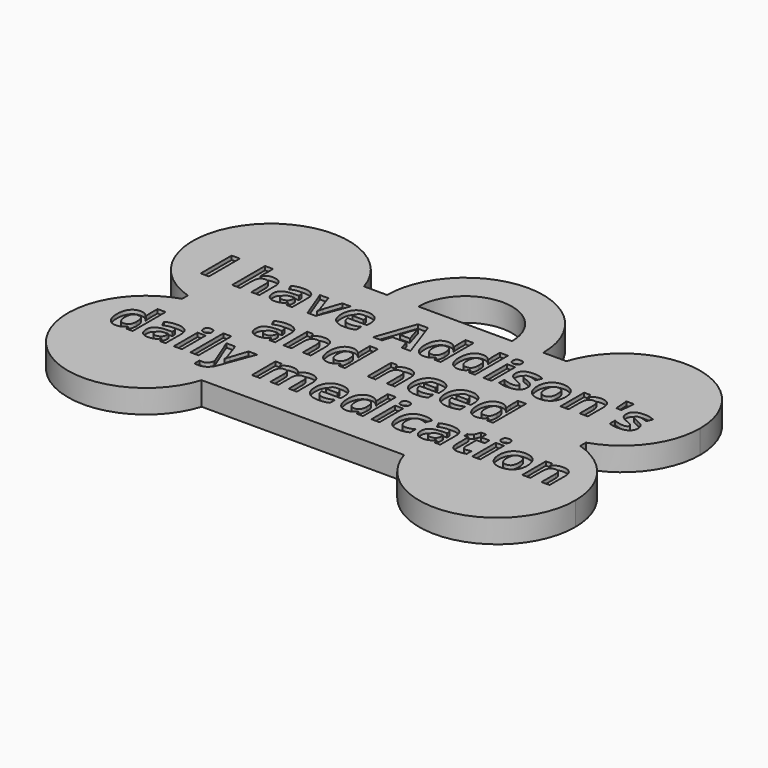
from build123d import *

# Parameters (mm, degrees)
F0_W          = 45
F0_H          = 20
F1_DEPTH      = 3
F3_DEPTH      = 3
F4_W          = 51
F4_H          = 26
F5_DEPTH      = 3
F6_R          = 10
F6_R_2        = 6
F7_DEPTH      = 3
F8_TEXT_SIZE  = 6.9444444444
F9_DEPTH      = 0.5
F10_TEXT_SIZE = 6.9444444444
F11_DEPTH     = 0.5


# Not quite as in the source:
# - Text() gives the source's letters only with a copy of the font that has no kerning and outlines rounded to 1/6400 em; it was checked with that copy


with BuildPart() as f1:
    # F0 (on Top) → F1 (new body)
    with BuildSketch(Plane.XY):
        with Locations((6.4884250968, 4.8540276475)):
            Rectangle(F0_W, F0_H)
    extrude(amount=F1_DEPTH)

    # F2 (on face) → F3 (join)
    with BuildSketch(Plane.XY.offset(3)):
        with BuildLine():
            ThreePointArc((28.9884250968, 4.8540276475), (36.0594929086, 7.7829598357), (38.9884250968, 14.8540276475))
            ThreePointArc((38.9884250968, 14.8540276475), (21.9173572849, 21.9250954594), (28.9884250968, 4.8540276475))
        make_face()
        with BuildLine():
            ThreePointArc((38.9884250968, -5.1459723525), (36.0594929086, 1.9250954594), (28.9884250968, 4.8540276475))
            ThreePointArc((28.9884250968, 4.8540276475), (21.9173572849, -12.2170401643), (38.9884250968, -5.1459723525))
        make_face()
        with BuildLine():
            ThreePointArc((-16.0115749032, 4.8540276475), (-23.0826427151, -12.2170401643), (-6.0115749032, -5.1459723525))
            ThreePointArc((-6.0115749032, -5.1459723525), (-8.9405070914, 1.9250954594), (-16.0115749032, 4.8540276475))
        make_face()
        with BuildLine():
            ThreePointArc((-6.0115749032, 14.8540276475), (-23.0826427151, 21.9250954594), (-16.0115749032, 4.8540276475))
            ThreePointArc((-16.0115749032, 4.8540276475), (-8.9405070914, 7.7829598357), (-6.0115749032, 14.8540276475))
        make_face()
    extrude(amount=-F3_DEPTH)

    # F4 (on face) → F5 (join)
    with BuildSketch(Plane.XY.offset(3)):
        with Locations((6.4884250968, 4.8540276475)):
            Rectangle(F4_W, F4_H)
    extrude(amount=-F5_DEPTH)

    # F6 (on face) → F7 (join)
    with BuildSketch(Plane.XY.offset(3)):
        with Locations((6.4884250968, 17.8540276475)):
            Circle(F6_R)
        with Locations((6.4884250968, 17.8540276475)):
            Circle(F6_R_2, mode=Mode.SUBTRACT)
    extrude(amount=-F7_DEPTH)

    # F8 (on face) → F9 (cut)
    with BuildSketch(Plane.XY.offset(3)):
        with Locations((-21.6224690004, 9.8540276475)):
            Text("I have Addison's", F8_TEXT_SIZE, font='Open Sans', font_style=FontStyle.BOLD, text_align=(TextAlign.LEFT, TextAlign.BOTTOM))
        with Locations((-9.5277424379, 2.8540276475)):
            Text('and need', F8_TEXT_SIZE, font='Open Sans', font_style=FontStyle.BOLD, text_align=(TextAlign.LEFT, TextAlign.BOTTOM))
        with Locations((-22.3662841046, -4.1459723525)):
            Text('daily medication', F8_TEXT_SIZE, font='Open Sans', font_style=FontStyle.BOLD, text_align=(TextAlign.LEFT, TextAlign.BOTTOM))
    extrude(amount=-F9_DEPTH, mode=Mode.SUBTRACT)

    # F10 (on face) → F11 (cut)
    with BuildSketch(Plane(origin=(0, 0, 0), x_dir=(1, 0, 0), z_dir=(0, 0, -1))):
        with Locations(Location((37.3570231871, -9.8540276475), (0, 0, 180))):
            Text('Please take me to', F10_TEXT_SIZE, font='Open Sans', font_style=FontStyle.BOLD, text_align=(TextAlign.LEFT, TextAlign.BOTTOM))
        with Locations(Location((26.6359945412, -2.8540276475), (0, 0, 180))):
            Text('the nearest', F10_TEXT_SIZE, font='Open Sans', font_style=FontStyle.BOLD, text_align=(TextAlign.LEFT, TextAlign.BOTTOM))
        with Locations(Location((35.683303569, 4.1459723525), (0, 0, 180))):
            Text('emergency clinic', F10_TEXT_SIZE, font='Open Sans', font_style=FontStyle.BOLD, text_align=(TextAlign.LEFT, TextAlign.BOTTOM))
    extrude(amount=-F11_DEPTH, mode=Mode.SUBTRACT)


solid = f1.part
